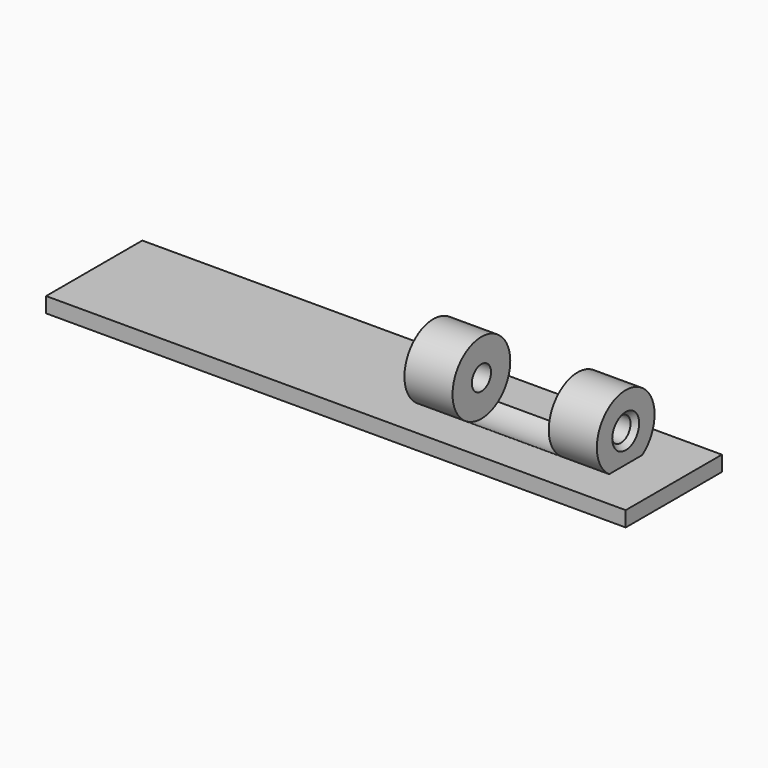
from build123d import *

# Parameters (mm, degrees)
F0_W      = 120.5
F0_H      = 3.175
F1_DEPTH  = 25
F2_R      = 7.5
F3_DEPTH  = 20
F4_R      = 7.5
F5_DEPTH  = 20
F6_R      = 7.5
F7_DEPTH  = 80.5
F8_W      = 26.1427015066
F8_H      = 14.1189814121
F9_DEPTH  = 70.5
F10_W     = 25
F10_H     = 14.862489751
F11_DEPTH = 10
F12_R     = 2.5
F13_DEPTH = 80
F15_DEPTH = 3
F16_SIZE  = 1


# Not quite as in the source:
# - a feature names something its author has since deleted; it is built from what else it names


with BuildPart() as f1:
    # F0 (on Front) → F1 (new body)
    with BuildSketch(Plane.XZ):
        Rectangle(F0_W, F0_H)
    extrude(amount=F1_DEPTH)

    # F2 (on face) → F3 (join)
    with BuildSketch(Plane.YZ.offset(60.25)):
        with Locations((-12.5, 7.7303019352)):
            Circle(F2_R)
    extrude(amount=-F3_DEPTH)

    # F4 (on face) → F5 (cut)
    with BuildSketch(Plane(origin=(40.25, 0, 0), x_dir=(0, -1, 0), z_dir=(-1, 0, 0))):
        with Locations((12.5, 7.7303019352)):
            Circle(F4_R)
    extrude(amount=F5_DEPTH, mode=Mode.SUBTRACT)

    # F6 (on face) → F7 (join)
    with BuildSketch(Plane(origin=(-60.25, 0, 0), x_dir=(0, -1, 0), z_dir=(-1, 0, 0))):
        with Locations((12.5, 7.7305)):
            Circle(F6_R)
    extrude(amount=-F7_DEPTH)

    # F8 (on face) → F9 (cut)
    with BuildSketch(Plane(origin=(-60.25, 0, 0), x_dir=(0, -1, 0), z_dir=(-1, 0, 0))):
        with Locations((13.0713507533, 8.646990706)):
            Rectangle(F8_W, F8_H)
    extrude(amount=-F9_DEPTH, mode=Mode.SUBTRACT)

    # F10 (on face) → F11 (cut)
    with BuildSketch(Plane.YZ.offset(60.25)):
        with Locations((-12.5, 9.0187448755)):
            Rectangle(F10_W, F10_H)
    extrude(amount=-F11_DEPTH, mode=Mode.SUBTRACT)

    # F12 (on face) → F13 (cut)
    with BuildSketch(Plane(origin=(10.25, 0, 0), x_dir=(0, -1, 0), z_dir=(-1, 0, 0))):
        with Locations((12.5, 7.7305)):
            Circle(F12_R)
    extrude(amount=-F13_DEPTH, mode=Mode.SUBTRACT)

    # F14 (on face) → F15 (cut)
    with BuildSketch(Plane(origin=(10.25, 0, 0), x_dir=(0, -1, 0), z_dir=(-1, 0, 0))):
        Polygon((12.5147298399, 4.3905242768), (15.3998687443, 6.0732685539), (15.3851389044, 9.4132442772), (12.4852701601, 11.0704757232), (9.6001312557, 9.3877314461), (9.6148610956, 6.0477557228), align=None)
    extrude(amount=-F15_DEPTH, mode=Mode.SUBTRACT)

    # F16
    f16_edges = [f1.edges().sort_by_distance(p)[0] for p in [
        (50.25, -10, 7.7305),
    ]]
    chamfer(f16_edges, length=F16_SIZE)


solid = f1.part
